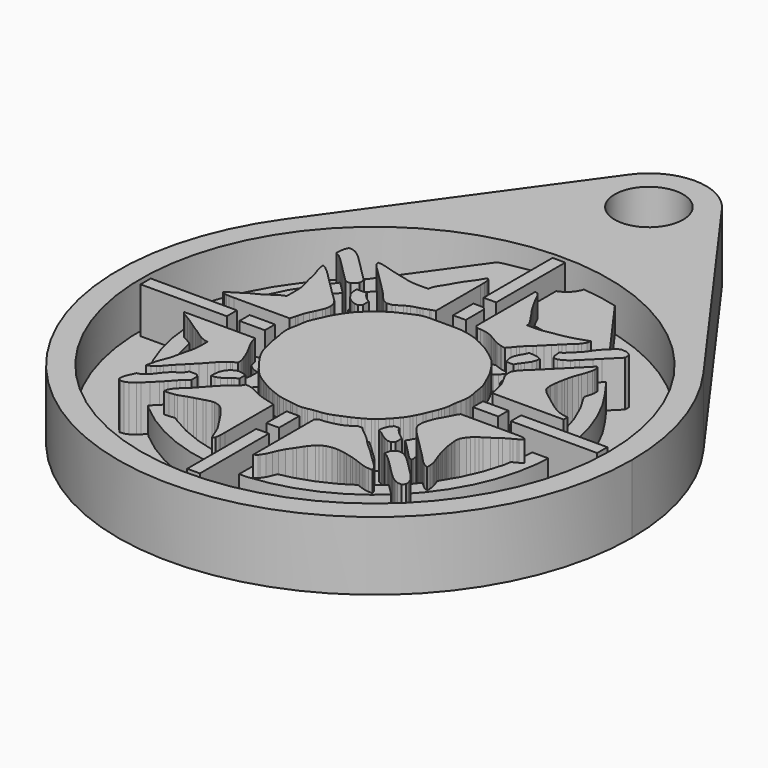
from build123d import *

# Parameters (mm, degrees)
F0_R     = 20.5
F0_R_2   = 3
F1_DEPTH = 6
F2_DEPTH = 2
F3_W     = 1.1111111111
F3_H     = 2.2222222222
F3_H_2   = 7.5555555556
F3_W_2   = 2.2222222222
F3_H_3   = 1.1111111111
F3_W_3   = 7.5555555556
F4_DEPTH = 4
F5_SCALE = 0.7


with BuildPart() as f1:
    # F0 (on Top) → F1 (new body)
    with BuildSketch(Plane.XY):
        with BuildLine():
            ThreePointArc((-18.2752393965, 13.125), (-6.894095792, -21.4177833403), (22.5, 0))
            ThreePointArc((22.5, 0), (21.4177833403, 6.894095792), (18.2752393965, 13.125))
            ThreePointArc((18.2752393965, 13.125), (0, 22.5), (-18.2752393965, 13.125))
        make_face()
        Circle(F0_R, mode=Mode.SUBTRACT)
        with BuildLine():
            ThreePointArc((-18.2752393965, 13.125), (0, 22.5), (18.2752393965, 13.125))
            Line((18.2752393965, 13.125), (4.0611643103, 32.9166666667))
            ThreePointArc((4.0611643103, 32.9166666667), (4.7595074089, 31.5320212871), (5, 30))
            ThreePointArc((5, 30), (-1.5320212871, 25.2404925911), (-4.0611643103, 32.9166666667))
            Line((-4.0611643103, 32.9166666667), (-18.2752393965, 13.125))
        make_face()
        with BuildLine():
            ThreePointArc((5, 30), (4.7595074089, 31.5320212871), (4.0611643103, 32.9166666667))
            ThreePointArc((4.0611643103, 32.9166666667), (0, 35), (-4.0611643103, 32.9166666667))
            ThreePointArc((-4.0611643103, 32.9166666667), (-1.5320212871, 25.2404925911), (5, 30))
        make_face()
        with Locations((0, 30)):
            Circle(F0_R_2, mode=Mode.SUBTRACT)
    extrude(amount=F1_DEPTH)

    # F0 (on Top) → F2 (join)
    with BuildSketch(Plane.XY):
        Circle(F0_R)
    extrude(amount=F2_DEPTH)

    # F3 (on face) → F4 (join)
    with BuildSketch(Plane.XY.offset(2)):
        Polygon((-1.7777777778, 7.7592586667), (-2.2222222222, 7.6728397778), (-2.6666666667, 7.5), (-2.8888888889, 7.3888888889), (-3.1111111111, 7.2962968889), (-3.3333333333, 7.1913588889), (-3.5555555556, 7.0987651111), (-4, 6.8703697778), (-4.4382713333, 6.592592), (-4.6481475556, 6.4444444444), (-5.0246922222, 6.1481475556), (-5.3827157778, 5.8456793333), (-5.7654317778, 5.5061731111), (-5.9506175556, 5.3148142222), (-6.1296293333, 5.104938), (-6.4444444444, 4.6666666667), (-6.5925928889, 4.4444444444), (-6.8703706667, 4), (-7.0987651111, 3.5555555556), (-7.191358, 3.3333333333), (-7.3888888889, 2.8888888889), (-7.5, 2.6666666667), (-7.6728397778, 2.2222222222), (-7.7654317778, 1.7777777778), (-7.7901237778, 1.5555555556), (-7.8641975556, 1.1111111111), (-7.9135802222, 0.8888888889), (-7.9814817778, 0.4444444444), (-7.9814817778, 0), (-7.9135802222, -0.4444444444), (-7.8641975556, -0.6666666667), (-7.7901237778, -1.1111111111), (-7.7654317778, -1.3333333333), (-7.691358, -1.7777777778), (-7.6358024444, -2), (-7.5246913333, -2.4444444444), (-7.4691357778, -2.6666666667), (-7.3271602222, -3.1111111111), (-7.2407413333, -3.3333333333), (-7.0185191111, -3.7777777778), (-6.8827157778, -4), (-6.5802468889, -4.4444444444), (-6.4135802222, -4.6666666667), (-6.0802468889, -5.1111111111), (-5.9135802222, -5.3333333333), (-5.5370364444, -5.7716046667), (-5.3271602222, -5.9814817778), (-4.8888888889, -6.3395064444), (-4.4444444444, -6.6234571111), (-4.2222222222, -6.7530864444), (-4, -6.8888888889), (-3.5555555556, -7.1358024444), (-3.1111111111, -7.3333333333), (-2.8888888889, -7.4197531111), (-2.4444444444, -7.5925928889), (-2.2222222222, -7.6728397778), (-1.7777777778, -7.7654317778), (-1.5555555556, -7.7901237778), (-1.1111111111, -7.8641975556), (-0.8888888889, -7.9135802222), (-0.4444444444, -7.9814817778), (0, -7.9814817778), (0.2222222222, -7.9506175556), (0.4444444444, -7.9135802222), (0.8888888889, -7.8271602222), (1.1111111111, -7.796296), (1.5555555556, -7.7592595556), (2, -7.6728397778), (2.2222222222, -7.5925928889), (2.4444444444, -7.512346), (2.8888888889, -7.3333333333), (3.3333333333, -7.1481484444), (3.5555555556, -7.0555555556), (4, -6.8395064444), (4.2160491111, -6.7160491111), (4.4259253333, -6.6111111111), (4.80247, -6.3580246667), (4.9753077778, -6.2160491111), (5.1604935556, -6.0679015556), (5.5432095556, -5.7283953333), (5.7283953333, -5.5432095556), (5.907408, -5.3456793333), (6.2160491111, -4.9753077778), (6.3580255556, -4.80247), (6.6111111111, -4.4259253333), (6.7160491111, -4.2160491111), (6.8395064444, -4), (7.0555555556, -3.5555555556), (7.1481475556, -3.3333333333), (7.3333333333, -2.8888888889), (7.512346, -2.4444444444), (7.592592, -2.2222222222), (7.6728397778, -2), (7.7592586667, -1.5555555556), (7.7962968889, -1.1111111111), (7.8271602222, -0.8888888889), (7.9135811111, -0.4444444444), (7.9814808889, 0), (7.9814808889, 0.4444444444), (7.9135811111, 0.8888888889), (7.8641966667, 1.1111111111), (7.7901237778, 1.5555555556), (7.7654317778, 1.7777777778), (7.6728397778, 2.2222222222), (7.5, 2.6666666667), (7.3888888889, 2.8888888889), (7.1913588889, 3.3333333333), (7.0987651111, 3.5555555556), (6.8703697778, 4), (6.592592, 4.4444444444), (6.4444444444, 4.6666666667), (6.2901237778, 4.8888888889), (5.9506175556, 5.3271602222), (5.7592586667, 5.5370364444), (5.3333333333, 5.9135811111), (5.1111111111, 6.0802477778), (4.6666666667, 6.407408), (4.4444444444, 6.5679015556), (4, 6.8333333333), (3.7777777778, 6.9382713333), (3.5555555556, 7.0617286667), (3.3333333333, 7.1604935556), (3.1111111111, 7.2777777778), (2.6666666667, 7.4567904444), (2.2222222222, 7.5864188889), (2, 7.6358033333), (1.7777777778, 7.6913588889), (1.3333333333, 7.7592586667), (1.1111111111, 7.7716046667), (0.6666666667, 7.7777777778), (0.2222222222, 7.7777777778), (-0.6666666667, 7.7777777778), (-1.1111111111, 7.7777777778), (-1.3333333333, 7.7777777778), align=None)
        Polygon((-8.8888888889, -2), (-15.1111111111, -2), (-14.9382713333, -2.2222222222), (-14.8209877778, -2.2716046667), (-14.4382713333, -2.5), (-14, -2.7654317778), (-13.5555555556, -3.0740746667), (-13.3333333333, -3.2345682222), (-12.8888888889, -3.5185191111), (-12.6666666667, -3.6543206667), (-12.2222222222, -3.9629635556), (-12, -4.1172842222), (-11.7901237778, -4.2345682222), (-11.4444444444, -4.3827157778), (-11.1111111111, -4.4444444444), (-11.1111111111, -4.9012348889), (-11.1172842222, -5.3333333333), (-11.1296293333, -5.5555555556), (-11.1975308889, -6), (-11.2530864444, -6.2222222222), (-11.3024691111, -6.4444444444), (-11.3641975556, -6.6666666667), (-11.4691357778, -7.1111111111), (-11.512346, -7.3333333333), (-11.6172842222, -7.7777777778), (-11.7777777778, -8.2222222222), (-11.8703706667, -8.4444444444), (-12.0246913333, -8.8888888889), (-12.0802468889, -9.0987651111), (-12.1666666667, -9.4444444444), (-12.2222222222, -9.7777777778), (-11.895062, -9.6604935556), (-11.5925928889, -9.4444444444), (-11.4197531111, -9.2777777778), (-11.2469135556, -9.0925928889), (-10.8703706667, -8.6666666667), (-10.6604935556, -8.4444444444), (-10.2222222222, -8), (-10, -7.7777777778), (-9.5617286667, -7.3333333333), (-9.1604935556, -6.895062), (-8.8024691111, -6.4938268889), (-8.6172842222, -6.308642), (-8.2283953333, -5.9753086667), (-8.012346, -5.8271602222), (-7.8888888889, -5.7222222222), (-7.5555555556, -5.5555555556), (-7.5740737778, -5.2222222222), (-7.6604935556, -4.8765428889), (-7.7407404444, -4.6666666667), (-7.8209873333, -4.4444444444), (-7.9197531111, -4.2222222222), (-8.012346, -4), (-8.2345682222, -3.5555555556), (-8.3641975556, -3.3333333333), (-8.604938, -2.8888888889), (-8.6975308889, -2.6790126667), (-8.8271602222, -2.3333333333), align=None)
        Polygon((-8.6666666667, -8.6666666667), (-9.3333333333, -8.6666666667), (-9.5061731111, -8.9753086667), (-9.6234571111, -9.0555555556), (-9.796296, -9.2098762222), (-9.987654, -9.3333333333), (-10.3580246667, -9.6234571111), (-10.6975308889, -10.0061731111), (-10.8580246667, -10.2222222222), (-11.1975308889, -10.6419753333), (-11.5617286667, -10.9506175556), (-11.6728397778, -11.0308642222), (-12, -11.1111111111), (-12.1481484444, -11.4444444444), (-12.2160491111, -11.5679015556), (-12.308642, -11.7777777778), (-12.4197531111, -12.1111111111), (-12.4444444444, -12.4444444444), (-12.2222222222, -12.6666666667), (-11.8888888889, -12.6419753333), (-11.5432095556, -12.5061731111), (-11.1111111111, -12.1975308889), (-10.8888888889, -11.9938268889), (-10.4444444444, -11.5555555556), (-10, -11.1111111111), (-9.7839508889, -10.8888888889), (-9.5740737778, -10.6666666667), (-9.1975308889, -10.2407404444), (-9.0370373333, -10.0617286667), (-8.7592586667, -9.796296), (-8.4444444444, -9.5555555556), (-8.4444444444, -8.8888888889), align=None)
        Polygon((-7.7716046667, -7.8888888889), (-7.7777777778, -8.2222222222), (-7.4444444444, -8.1975308889), (-7.0987651111, -8.0617286667), (-6.6790126667, -7.7777777778), (-6.4567904444, -7.6172842222), (-6.3333333333, -7.5061731111), (-6, -7.3333333333), (-6, -6.6666666667), (-6.4567904444, -6.5432095556), (-6.6790126667, -6.5185191111), (-6.8827157778, -6.5370373333), (-7.2777777778, -6.7407413333), (-7.5679015556, -7.1172842222), (-7.6666666667, -7.3333333333), (-7.7222222222, -7.5432095556), align=None)
        Polygon((-4.7777777778, -7.796296), (-5.1111111111, -7.7777777778), (-5.2839508889, -8.092592), (-5.4012348889, -8.1790126667), (-5.5740746667, -8.3518515556), (-5.7654317778, -8.4814817778), (-6.1358024444, -8.7716046667), (-6.308642, -8.9444444444), (-6.6851848889, -9.3395064444), (-7.0925928889, -9.7777777778), (-7.4691357778, -10.203704), (-7.6419753333, -10.395062), (-7.8271602222, -10.5802468889), (-8.2222222222, -10.9382713333), (-8.4197531111, -11.1296293333), (-8.592592, -11.3271602222), (-8.808642, -11.6666666667), (-8.8888888889, -12), (-8.4320984444, -11.9938268889), (-8, -11.9444444444), (-7.7777777778, -11.895062), (-7.3333333333, -11.7407404444), (-7.1111111111, -11.6543206667), (-6.6666666667, -11.5246913333), (-6.4444444444, -11.4691357778), (-6, -11.3333333333), (-5.7777777778, -11.2654317778), (-5.3333333333, -11.1666666667), (-5.1111111111, -11.1543206667), (-4.6728397778, -11.2716046667), (-4.4629635556, -11.407408), (-4.2716046667, -11.5802468889), (-4.0864188889, -11.7839508889), (-3.7469144444, -12.2222222222), (-3.4320984444, -12.6666666667), (-3.2962968889, -12.8888888889), (-3.012346, -13.3333333333), (-2.8580255556, -13.5555555556), (-2.5802477778, -14), (-2.3765428889, -14.4444444444), (-2.30247, -14.6543211111), (-2.2160491111, -14.8765433333), (-2.1790126667, -15), (-2, -15.3333333333), (-1.8395064444, -15.1604935556), (-1.8333333333, -15.04321), (-1.7901237778, -14.8641975556), (-1.7839508889, -14.6604935556), (-1.7777777778, -14.2222222222), (-1.7777777778, -14), (-1.7777777778, -13.3333333333), (-1.7777777778, -8.8888888889), (-2.2345682222, -8.7530864444), (-2.6666666667, -8.6358024444), (-2.8888888889, -8.5802468889), (-3.3333333333, -8.4259262222), (-3.7777777778, -8.2098762222), (-4, -8.0864197778), (-4.4320984444, -7.8888888889), align=None)
        with Locations((0.1111111111, -10.2222222222)):
            Rectangle(F3_W, F3_H)
        with Locations((0.1111111111, -16.2222222222)):
            Rectangle(F3_W, F3_H_2)
        Polygon((5.1111111111, -7.7777777778), (4.6666666667, -7.7777777778), (4.3333333333, -8.0493824444), (3.987654, -8.2469135556), (3.7777777778, -8.3395064444), (3.3333333333, -8.4753086667), (2.8888888889, -8.5802468889), (2.4567904444, -8.6481484444), (2.3333333333, -8.6604935556), (2, -8.6666666667), (1.7777777778, -8.8888888889), (1.7777777778, -15.5555555556), (2.0493824444, -15.3827157778), (2.1296284444, -15.2654322222), (2.3827157778, -14.8827157778), (2.5802477778, -14.4444444444), (2.7592604444, -14), (2.9938268889, -13.5555555556), (3.2962968889, -13.1111111111), (3.4567904444, -12.8888888889), (3.7407413333, -12.4444444444), (3.8827157778, -12.2283953333), (4.2407413333, -11.8333333333), (4.4506175556, -11.6666666667), (4.6666666667, -11.5432095556), (4.8888888889, -11.4444444444), (5.3333333333, -11.3518515556), (5.7777777778, -11.3395064444), (6, -11.3518515556), (6.4444444444, -11.4197531111), (6.6666666667, -11.4753086667), (7.1111111111, -11.5864197778), (7.3333333333, -11.6419753333), (7.7777777778, -11.7839508889), (8.2222222222, -11.9567904444), (8.6666666667, -12.1172842222), (8.8765428889, -12.1666666667), (9.2222222222, -12.2160491111), (9.5555555556, -12.2222222222), (9.4382731111, -11.907408), (9.3518542222, -11.8148151111), (9.2222222222, -11.6296293333), (8.8703715556, -11.2839508889), (8.6604953333, -11.0925928889), (8.2222222222, -10.6666666667), (8, -10.4444444444), (7.5555555556, -10.0185182222), (7.3395064444, -9.8271602222), (6.9382713333, -9.4691357778), (6.7530855556, -9.2839508889), (6.395062, -8.9012348889), (6.2037031111, -8.7160491111), (5.7901237778, -8.3703706667), (5.5679015556, -8.1851848889), (5.4444444444, -8.092592), align=None)
        Polygon((7.1111111111, -6.2222222222), (6.6666666667, -6.2222222222), (6.4135811111, -6.5555555556), (6.3703697778, -6.6666666667), (6.2469144444, -7), (6.2222222222, -7.3333333333), (6.5555555556, -7.5061731111), (6.6790126667, -7.6172842222), (6.9012348889, -7.7777777778), (7.3209873333, -8.0617286667), (7.6666666667, -8.1975308889), (8, -8.2222222222), (8.2222222222, -8), (8.2222222222, -7.3333333333), (7.9074062222, -7.0987651111), (7.6358033333, -6.8765428889), (7.4938268889, -6.7469135556), (7.3518524444, -6.5864197778), (7.2654317778, -6.5), align=None)
        Polygon((8.7407431111, -9.3456793333), (8.6666666667, -9.7777777778), (9, -9.9506175556), (9.1234571111, -10.0679015556), (9.3456793333, -10.2469135556), (9.5555555556, -10.4506175556), (9.7777777778, -10.6666666667), (10, -10.8888888889), (10.4444444444, -11.3333333333), (10.8888888889, -11.7777777778), (11.1111111111, -11.9938268889), (11.3333333333, -12.1975308889), (11.7654317778, -12.5061731111), (12.1111111111, -12.6419753333), (12.4444444444, -12.6666666667), (12.6666666667, -12.4444444444), (12.6419744444, -12.1111111111), (12.5061713333, -11.7654317778), (12.19753, -11.3333333333), (11.9938286667, -11.1111111111), (11.7777777778, -10.8888888889), (11.3333333333, -10.4444444444), (10.8888888889, -10), (10.6666666667, -9.7777777778), (10.2222222222, -9.3580246667), (9.7777777778, -9.0493824444), (9.5555555556, -8.9691357778), (9.3395046667, -8.9382713333), (9.1358033333, -8.9691357778), (8.827162, -9.1728397778), align=None)
        Polygon((12.8888888889, -2), (9.1111111111, -2), (8.8888888889, -2.3333333333), (8.8395046667, -2.4567904444), (8.6111111111, -2.8888888889), (8.3641966667, -3.3333333333), (8.2407413333, -3.5555555556), (8.1358033333, -3.7777777778), (7.9753077778, -4.2222222222), (7.9197522222, -4.4444444444), (7.8703697778, -4.6666666667), (7.8703697778, -5.1111111111), (7.9444444444, -5.3333333333), (8.0740728889, -5.5555555556), (8.4506157778, -6), (8.6666666667, -6.2222222222), (9.1111111111, -6.6666666667), (9.5555555556, -7.1111111111), (10.2222222222, -7.7777777778), (10.6666666667, -8.2222222222), (11.0925937778, -8.6604935556), (11.2839491111, -8.8703706667), (11.6296284444, -9.2222222222), (11.814816, -9.3518524444), (11.9074097778, -9.4382713333), (12.2222222222, -9.5555555556), (12.2160508889, -9.2222222222), (12.1666666667, -8.8765428889), (12.1172824444, -8.6666666667), (11.9567904444, -8.2222222222), (11.7839491111, -7.7777777778), (11.6419744444, -7.3333333333), (11.5864188889, -7.1111111111), (11.4753077778, -6.6666666667), (11.4197522222, -6.4444444444), (11.3827175556, -6.2222222222), (11.3209873333, -5.7777777778), (11.2716064444, -5.3333333333), (11.3209873333, -4.8888888889), (11.5864188889, -4.4506175556), (11.7839491111, -4.2407413333), (12, -4.0555555556), (12.2222222222, -3.8827157778), (12.4444444444, -3.7407413333), (12.8888888889, -3.4567904444), (13.3333333333, -3.1481475556), (13.5555555556, -2.987654), (14, -2.7222222222), (14.2098762222, -2.6234571111), (14.4320984444, -2.4938268889), (14.5555555556, -2.4444444444), (14.8888888889, -2.2222222222), (14.7160508889, -2.0617286667), (14.5987651111, -2.0555555556), (14.4197522222, -2.012346), (14.2160508889, -2.0061731111), (13.7777777778, -2), (13.5555555556, -2), align=None)
        with Locations((10.2222222222, -0.1111111111)):
            Rectangle(F3_W_2, F3_H_3)
        with Locations((16.2222222222, -0.1111111111)):
            Rectangle(F3_W_3, F3_H_3)
        Polygon((12.1543206667, 9.1604953333), (12, 9.3333333333), (10, 7.3333333333), (9.3333333333, 6.6666666667), (9.1111111111, 6.4444444444), (8.672838, 6.0185191111), (8.2777777778, 5.6419744444), (8.1111111111, 5.4691366667), (7.895062, 5.092592), (7.8518524444, 4.8827157778), (7.895062, 4.4444444444), (7.9814826667, 4.2222222222), (8.2222222222, 3.7777777778), (8.4629617778, 3.3333333333), (8.5555555556, 3.1111111111), (8.6172824444, 2.8888888889), (8.7098762222, 2.4567904444), (8.7592604444, 2.2345682222), (8.8888888889, 1.7777777778), (15.1111111111, 1.7777777778), (15.1111111111, 2.2222222222), (14.7777777778, 2.2407413333), (14.4320984444, 2.3271602222), (14, 2.5061731111), (13.5555555556, 2.7654317778), (13.3333333333, 2.9259253333), (12.8888888889, 3.2530855556), (12.6666666667, 3.4135811111), (12.4444444444, 3.5864188889), (12, 3.9197522222), (11.7839491111, 4.0864188889), (11.4259271111, 4.4629635556), (11.3209873333, 4.6728397778), (11.2716064444, 5.1111111111), (11.3209873333, 5.5555555556), (11.3456793333, 5.7777777778), (11.4197522222, 6.2222222222), (11.4691366667, 6.4444444444), (11.512346, 6.6666666667), (11.6172824444, 7.1111111111), (11.7777777778, 7.5555555556), (11.8703715556, 7.7777777778), (12.0246922222, 8.2222222222), (12.1296284444, 8.6604953333), (12.160492, 8.8641966667), (12.1481457778, 9.0432095556), align=None)
        Polygon((7.5555555556, 7.987654), (7.1111111111, 8), (6.9567904444, 7.6666666667), (6.7530873333, 7.3209873333), (6.5740746667, 6.8888888889), (6.5493824444, 6.6790126667), (6.5555555556, 6.4567904444), (6.6666666667, 6), (7.3333333333, 6), (7.5061731111, 6.3333333333), (7.6172842222, 6.4567904444), (7.7777777778, 6.6790126667), (8.0617286667, 7.0987651111), (8.19753, 7.4444444444), (8.2222222222, 7.7777777778), (7.8888888889, 7.9382713333), (7.7777777778, 7.9444444444), align=None)
        Polygon((8.9814791111, 9.5061713333), (8.6666666667, 9.3333333333), (8.7222222222, 8.8888888889), (8.7283968889, 8.7654317778), (8.8888888889, 8.4444444444), (9.2222222222, 8.4691366667), (9.5679015556, 8.6049397778), (10, 8.9135811111), (10.2222222222, 9.1172824444), (10.4444444444, 9.3333333333), (10.8888888889, 9.7777777778), (11.1111111111, 10), (11.5555555556, 10.4444444444), (12.6666666667, 11.5555555556), (12.6666666667, 12), (12.3333333333, 12.2530855556), (12.2098762222, 12.2901237778), (11.7839491111, 12.3456793333), (11.5740728889, 12.2777777778), (11.3827175556, 12.1543206667), (11.0246922222, 11.8209873333), (10.8456793333, 11.6419744444), (10.5061713333, 11.2839491111), (10.2222222222, 10.8888888889), (10.0864188889, 10.685184), (9.9382731111, 10.4938286667), (9.7716064444, 10.3086411111), (9.4197522222, 9.9567904444), (9.0740728889, 9.6172824444), align=None)
        Polygon((2.0370364444, 15.2530855556), (1.7777777778, 15.3333333333), (1.7777777778, 8.8888888889), (2, 8.6666666667), (2.3333333333, 8.6604953333), (2.6790126667, 8.6172824444), (2.8888888889, 8.5740728889), (3.1111111111, 8.5061713333), (3.3333333333, 8.4197522222), (3.5555555556, 8.3086411111), (4, 8.0432095556), (4.2222222222, 7.9135811111), (4.4444444444, 7.80247), (4.8765428889, 7.6481475556), (5, 7.6111111111), (5.3333333333, 7.5555555556), (5.6111111111, 7.8827157778), (5.8580255556, 8.1851857778), (6, 8.3518506667), (6.3148142222, 8.6666666667), (6.6666666667, 8.9814826667), (6.8456793333, 9.1543206667), (7.19753, 9.512346), (7.5555555556, 9.8641966667), (7.9135811111, 10.2222222222), (8.0864188889, 10.4012348889), (8.2716046667, 10.5802477778), (8.6666666667, 10.9382731111), (8.8641966667, 11.1296284444), (9.0370346667, 11.327162), (9.2530855556, 11.6666666667), (9.3333333333, 12), (9, 11.9012348889), (8.8765428889, 11.8518506667), (8.6543206667, 11.7777777778), (8.2222222222, 11.6419744444), (8, 11.5864188889), (7.7777777778, 11.5246922222), (7.3333333333, 11.4197522222), (6.8888888889, 11.3456793333), (6.6666666667, 11.3209873333), (6.4444444444, 11.2839491111), (6.2222222222, 11.2469144444), (6, 11.19753), (5.5555555556, 11.1296284444), (5.3333333333, 11.1172824444), (4.9012348889, 11.1111111111), (4.4444444444, 11.1111111111), (4.3641984444, 11.4444444444), (4.2901237778, 11.5679015556), (4.1666666667, 11.7901237778), (3.8765428889, 12.2160508889), (3.7407413333, 12.4259271111), (3.4753077778, 12.80247), (3.3456793333, 12.9753077778), (3.1111111111, 13.3518506667), (2.8765428889, 13.7777777778), (2.7469144444, 14), (2.5061731111, 14.4444444444), (2.30247, 14.8641966667), (2.2160491111, 15.0370346667), (2.092592, 15.172838), align=None)
        Polygon((0.4444444444, 11.3333333333), (-0.4444444444, 11.3333333333), (-0.4444444444, 9.1111111111), (0.6666666667, 9.1111111111), (0.6666666667, 11.1111111111), align=None)
        with Locations((0.1111111111, 16.2222222222)):
            Rectangle(F3_W, F3_H_2)
        Polygon((-1.8395064444, 14.7160508889), (-2, 14.8888888889), (-2.2222222222, 14.5555555556), (-2.2777777778, 14.4382731111), (-2.5308633333, 14.0493842222), (-2.80247, 13.6913588889), (-3.0679015556, 13.314816), (-3.1913588889, 13.1049397778), (-3.3209873333, 12.8888888889), (-3.5555555556, 12.4629617778), (-3.7901237778, 12.0864188889), (-4.0185173333, 11.7407395556), (-4.1604935556, 11.4382697778), (-4.2222222222, 11.1111111111), (-4.9012348889, 11.1111111111), (-5.1111111111, 11.1111111111), (-5.5555555556, 11.1296284444), (-6, 11.19753), (-6.2222222222, 11.2530855556), (-6.6666666667, 11.3641966667), (-6.8888888889, 11.4135811111), (-7.1111111111, 11.4753077778), (-7.3333333333, 11.5246922222), (-7.7777777778, 11.6419744444), (-8, 11.7098762222), (-8.4444444444, 11.8456793333), (-8.6543206667, 11.9074062222), (-9, 11.9814826667), (-9.3333333333, 12), (-9.2530864444, 11.7222222222), (-9.1728397778, 11.6296284444), (-9.0370364444, 11.4567904444), (-8.6604935556, 11.0925937778), (-8.2222222222, 10.6666666667), (-7.7777777778, 10.2222222222), (-7.1111111111, 9.5555555556), (-6.6666666667, 9.1111111111), (-6.4506175556, 8.8888888889), (-6.2407404444, 8.6666666667), (-5.8641975556, 8.2283953333), (-5.6913588889, 8.0246922222), (-5.5061731111, 7.8518506667), (-5.104938, 7.6543206667), (-4.6666666667, 7.7160491111), (-4.4444444444, 7.8333333333), (-4, 8.1172842222), (-3.7777777778, 8.2345682222), (-3.5555555556, 8.3395064444), (-3.1111111111, 8.4753077778), (-2.8888888889, 8.5308633333), (-2.6666666667, 8.5987651111), (-2.2345682222, 8.7407395556), (-2.1111111111, 8.7901237778), (-1.7777777778, 8.8888888889), (-1.7777777778, 12.8888888889), (-1.7777777778, 13.5555555556), (-1.7777777778, 13.7777777778), (-1.7839508889, 14.2160508889), (-1.7901237778, 14.4197522222), (-1.8333333333, 14.5987651111), align=None)
        Polygon((-7.1111111111, 8), (-8, 8), (-7.9753086667, 7.5432095556), (-7.9259253333, 7.3209873333), (-7.8395064444, 7.1111111111), (-7.5308642222, 6.6913588889), (-7.1234571111, 6.3827157778), (-6.7777777778, 6.2469144444), (-6.4444444444, 6.2222222222), (-6.2222222222, 6.4444444444), (-6.2222222222, 7.1111111111), (-6.5, 7.2654317778), (-6.5864197778, 7.3518524444), (-6.7407404444, 7.4814808889), (-6.9567904444, 7.7222222222), align=None)
        Polygon((-11.8888888889, 12.4197522222), (-12.2222222222, 12.4444444444), (-12.3827157778, 12.1111111111), (-12.3888888889, 12), (-12.4320984444, 11.7777777778), (-12.4444444444, 11.3333333333), (-12.1111111111, 11.1604953333), (-11.987654, 11.0432095556), (-11.7654317778, 10.8641966667), (-11.5555555556, 10.6604953333), (-11.3333333333, 10.4444444444), (-10.8888888889, 10), (-10.4444444444, 9.5555555556), (-9.3333333333, 8.4444444444), (-8.8888888889, 8.4444444444), (-8.4444444444, 8.8888888889), (-8.4444444444, 9.3333333333), (-9.5555555556, 10.4444444444), (-10, 10.8888888889), (-10.2222222222, 11.1111111111), (-10.6666666667, 11.5555555556), (-10.8888888889, 11.7716064444), (-11.1111111111, 11.9753077778), (-11.5432095556, 12.2839491111), align=None)
        Polygon((-11.6666666667, 9.1604953333), (-12, 9.3333333333), (-11.9814817778, 9), (-11.895062, 8.6543206667), (-11.7407404444, 8.2222222222), (-11.6604935556, 8), (-11.5555555556, 7.5555555556), (-11.4629626667, 7.1111111111), (-11.4012348889, 6.8888888889), (-11.2654317778, 6.4444444444), (-11.203704, 6.2222222222), (-11.1296293333, 5.7777777778), (-11.1111111111, 5.3333333333), (-11.1111111111, 5.1111111111), (-11.1111111111, 4.9012348889), (-11.1111111111, 4.2222222222), (-11.4444444444, 4.104938), (-11.5679015556, 4.0185173333), (-11.7901237778, 3.895062), (-12.2222222222, 3.592592), (-12.4444444444, 3.4382713333), (-12.8888888889, 3.1975317778), (-13.3333333333, 2.9753077778), (-13.7777777778, 2.69753), (-14, 2.5432095556), (-14.4320988889, 2.2777777778), (-14.5555555556, 2.2222222222), (-14.8888888889, 2), (-14.7160491111, 1.8395064444), (-14.5987655556, 1.8333333333), (-14.4197531111, 1.7901237778), (-14.2160491111, 1.7839508889), (-13.7777777778, 1.7777777778), (-13.5555555556, 1.7777777778), (-12.8888888889, 1.7777777778), (-8.8888888889, 1.7777777778), (-8.7530864444, 2.2345682222), (-8.6975308889, 2.4567904444), (-8.5679015556, 2.8888888889), (-8.3888888889, 3.3333333333), (-8.2716046667, 3.5555555556), (-8.1728397778, 3.7777777778), (-7.9691357778, 4.2222222222), (-7.8827157778, 4.4444444444), (-7.8148151111, 4.8888888889), (-7.8888888889, 5.3148142222), (-8.1111111111, 5.6913588889), (-8.4629626667, 6.0493824444), (-8.6728397778, 6.2407413333), (-8.8888888889, 6.4506175556), (-9.1111111111, 6.6666666667), (-9.5555555556, 7.1111111111), (-10.2222222222, 7.7777777778), (-10.4444444444, 8), (-10.8888888889, 8.4444444444), (-11.1111111111, 8.6604953333), (-11.3209873333, 8.8641966667), (-11.5432095556, 9.0432095556), align=None)
        with Locations((-10.2222222222, -0.1111111111)):
            Rectangle(F3_W_2, F3_H_3)
        with Locations((-16.2222222222, -0.1111111111)):
            Rectangle(F3_W_3, F3_H_3)
    extrude(amount=F4_DEPTH)


with BuildPart() as f5_1:
    # F5: copy of F1
    add(f1.part.scale(F5_SCALE))


solid = Compound([f1.part, f5_1.part])
